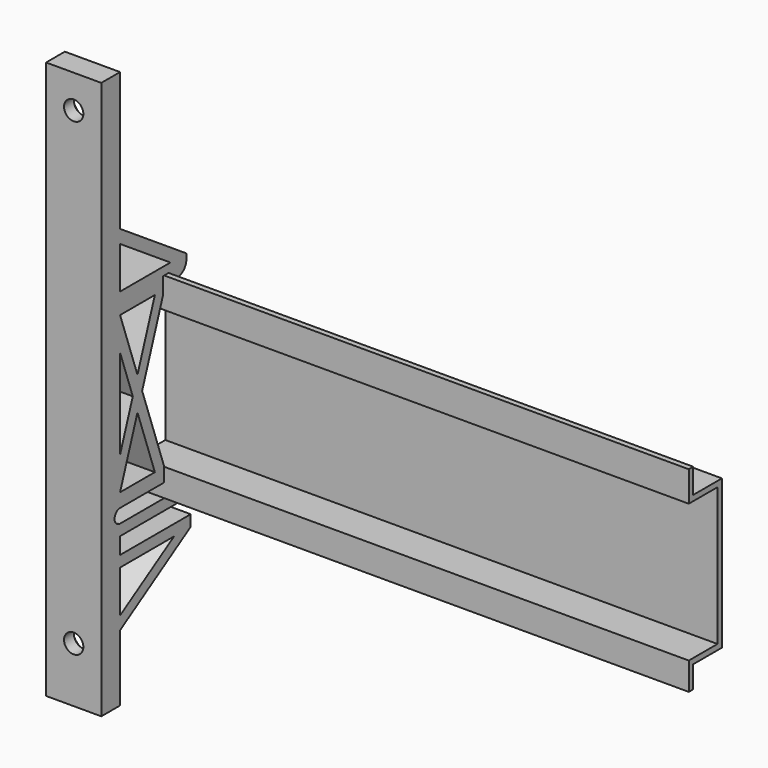
from build123d import *

# Parameters (mm, degrees)
F1_DEPTH       = 100
F2_W           = 4.25
F2_H           = 12
F3_DEPTH       = 5
F5_D           = 3.5
F5_CBORE_D     = 7.5
F5_CBORE_DEPTH = 17


# Not quite as in the source:
# - a feature names something its author has since deleted; it is built from what else it names


with BuildPart() as f1:
    # F0 (on Right) → F1 (new body)
    with BuildSketch(Plane.YZ):
        Polygon((-5.5, 18), (-6.5, 18), (-6.5, 12.5), (0, 12.5), (0, -12.5), (-6.5, -12.5), (-6.5, -17.5), (-5.5, -17.5), (-5.5, -13.5), (1, -13.5), (1, 13.5), (-5.5, 13.5), align=None)
    extrude(amount=F1_DEPTH)


with BuildPart() as f3:
    # F2 (on Right) → F3 (new body, symmetric)
    with BuildSketch(Plane.YZ):
        with BuildLine():
            ThreePointArc((-3.5, 16.5), (-2.0857864376, 17.0857864376), (-1.5, 18.5))
            Line((-1.5, 18.5), (-1.5, 19.5))
            Line((-1.5, 19.5), (-5.1055512755, 19.5))
            Line((-5.1055512755, 19.5), (-16.5, 19.5))
            Line((-16.5, 19.5), (-20.75, 19.5))
            Line((-20.75, 19.5), (-20.75, -19.5))
            Line((-20.75, -19.5), (-16.5, -19.5))
            Line((-16.5, -19.5), (-0.5, -19.5))
            Line((-0.5, -19.5), (-0.5, -19))
            Line((-0.5, -19), (-4.7132688278, -16.0507118205))
            ThreePointArc((-4.7132688278, -16.0507118205), (-5.2309051904, -16.0168384426), (-5.5, -16.4603277808))
            Line((-5.5, -16.4603277808), (-5.5, -17.5))
            Line((-5.5, -17.5), (-16.5, -17.5))
            ThreePointArc((-16.5, -17.5), (-17.75, -16.25), (-16.5, -15))
            Line((-16.5, -15), (-6.5, -15))
            Line((-6.5, -15), (-6.5, -12.5))
            Line((-6.5, -12.5), (-11.5, 1.625))
            Line((-11.5, 1.625), (-6.8, 14.9025))
            Line((-6.8, 14.9025), (-6.8, 18))
            Line((-6.8, 18), (-6.5, 18))
            Line((-6.5, 18), (-5.5, 18))
            Line((-5.5, 18), (-5.5, 17.5))
            ThreePointArc((-5.5, 17.5), (-5.2071067812, 16.7928932188), (-4.5, 16.5))
            Line((-4.5, 16.5), (-3.5, 16.5))
        make_face()
        Polygon((-16.5, -12.5), (-12.560803219, -1.3717690935), (-8.6216064379, -12.5), align=None, mode=Mode.SUBTRACT)
        Polygon((-12.560803219, 4.6217690935), (-11.5, 1.625), (-12.560803219, -1.3717690935), (-12.6095014243, -1.2341966635), (-13.6216064379, 1.625), (-16.5, -6.5064618129), (-16.5, 9.7564618129), (-16.5, 15.75), (-8.6216064379, 15.75), align=None, mode=Mode.SUBTRACT)
        Polygon((-16.5, -19.5), (-20.75, -19.5), (-20.75, -34.5), (-16.5, -34.5), (-0.5, -24.5), (-0.5, -22.5), (-16.5, -22.5), align=None)
        Polygon((-16.5, -32.141504717), (-16.5, -24.5), (-4.2735924528, -24.5), align=None, mode=Mode.SUBTRACT)
        Polygon((-16.5, 27.0962991497), (-16.5, 29.5), (-16.5, 54.5), (-20.75, 54.5), (-20.75, 19.5), (-16.5, 19.5), align=None)
        with Locations((-18.625, -40.5)):
            Rectangle(F2_W, F2_H)
        Polygon((-5.1055512755, 19.5), (-1.5, 19.5), (-16.5, 29.5), (-16.5, 27.0962991497), align=None)
        Polygon((-12.560803219, -1.3717690935), (-11.5, 1.625), (-12.560803219, 4.6217690935), (-16.5, 15.75), (-16.5, 9.7564618129), (-13.6216064379, 1.625), (-12.6095014243, -1.2341966635), align=None)
    extrude(amount=F3_DEPTH, both=True)

    # F5 (through all)
    with Locations(Plane(origin=(0, -1.5, 0), x_dir=(-1, 0, 0), z_dir=(0, 1, 0))):
        with Locations((0, 48.5), (0, -36.5)):
            CounterBoreHole(F5_D / 2, F5_CBORE_D / 2, F5_CBORE_DEPTH)


solid = Compound([f1.part, f3.part])
